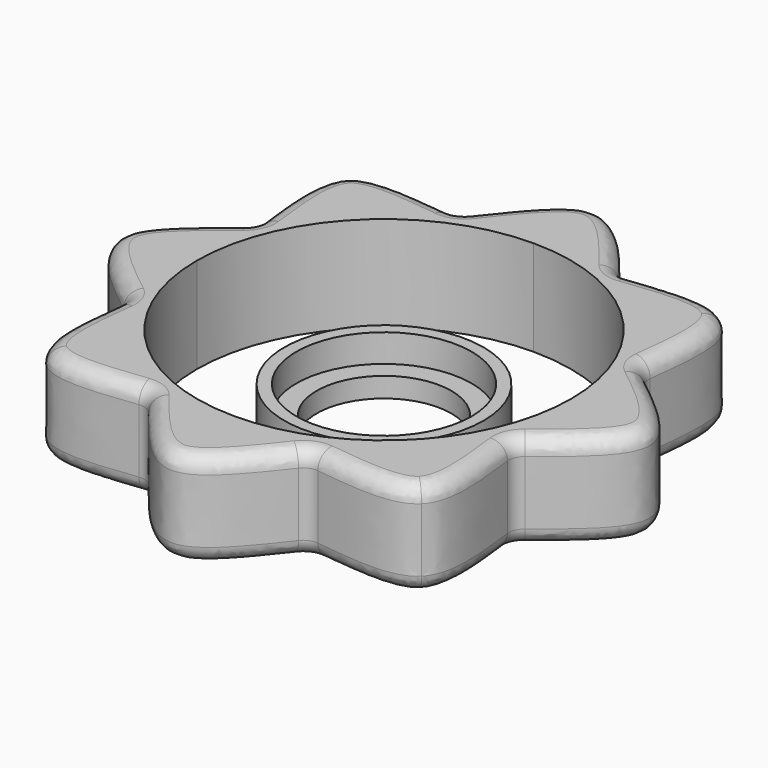
from build123d import *

# Parameters (mm, degrees)
F0_R     = 12.5
F0_R_2   = 11
F0_R_3   = 8.4561388704
F1_DEPTH = 2.5
F2_DEPTH = 12
F3_R     = 2
F4_DEPTH = 6


with BuildPart() as f1:
    # F0 (on Top) → F1 (new body)
    with BuildSketch(Plane.XY):
        Circle(F0_R)
        Circle(F0_R_2, mode=Mode.SUBTRACT)
        Circle(F0_R_2)
        Circle(F0_R_3, mode=Mode.SUBTRACT)
    extrude(amount=F1_DEPTH)

    # F0 (on Top) → F4 (join)
    with BuildSketch(Plane.XY):
        Circle(F0_R)
        Circle(F0_R_2, mode=Mode.SUBTRACT)
    extrude(amount=F4_DEPTH)


with BuildPart() as f2:
    # F0 (on Top) → F2 (new body)
    with BuildSketch(Plane.XY):
        with BuildLine():
            ThreePointArc((-23.5, 0), (-16.6170093579, 16.6170093579), (0, 23.5))
            add(Edge.make_bspline(
                [(-9.1409899994, 24.1728679287), (-6.2252758284, 23.8233956703), (-3.1123029045, 23.4999993166), (0, 23.5)],
                knots=[0.9614800765, 0.9614800765, 0.9614800765, 0.9614800765, 1, 1, 1, 1], degree=3))
            Line((-9.1409899994, 24.1728679287), (-16.656928964, 16.656928964))
            Line((-16.656928964, 16.656928964), (-24.1728340356, 9.1410238925))
            add(Edge.make_bspline(
                [(-23.5, 0), (-23.5, 3.1128517111), (-23.8233482549, 6.2257034223), (-24.1728340356, 9.1410238925)],
                knots=[0.7499999103, 0.7499999103, 0.7499999103, 0.7499999103, 0.7885112511, 0.7885112511, 0.7885112511, 0.7885112511], degree=3))
        make_face()
        with BuildLine():
            add(Edge.make_bspline(
                [(0, -23.5), (-3.1123029045, -23.4999993166), (-6.2252758284, -23.8233956703), (-9.1409899994, -24.1728679287)],
                knots=[0.4999998205, 0.4999998205, 0.4999998205, 0.4999998205, 0.538519744, 0.538519744, 0.538519744, 0.538519744], degree=3))
            ThreePointArc((0, -23.5), (-16.6170093579, -16.6170093579), (-23.5, 0))
            add(Edge.make_bspline(
                [(-24.1728340356, -9.1410238925), (-23.8233482549, -6.2257034223), (-23.5, -3.1128517111), (-23.5, 0)],
                knots=[0.7114885694, 0.7114885694, 0.7114885694, 0.7114885694, 0.7499999103, 0.7499999103, 0.7499999103, 0.7499999103], degree=3))
            Line((-24.1728340356, -9.1410238925), (-16.656928964, -16.656928964))
            Line((-16.656928964, -16.656928964), (-9.1409899994, -24.1728679287))
        make_face()
        with BuildLine():
            ThreePointArc((0, 23.5), (16.6170093579, 16.6170093579), (23.5, 0))
            ThreePointArc((23.5, 0), (16.6170093579, -16.6170093579), (0, -23.5))
            add(Edge.make_bspline(
                [(9.1406888631, -24.173169065), (6.2257012261, -23.8235819149), (3.1131858129, -23.5000006836), (0, -23.5)],
                knots=[0.4614689696, 0.4614689696, 0.4614689696, 0.4614689696, 0.4999998205, 0.4999998205, 0.4999998205, 0.4999998205], degree=3))
            Line((9.1406888631, -24.173169065), (16.656928964, -16.656928964))
            Line((16.656928964, -16.656928964), (24.214399877, -9.0994580511))
            add(Edge.make_bspline(
                [(23.5564548484, 0), (23.5564548484, -3.0980623812), (23.8727564423, -6.1961247624), (24.214399877, -9.0994580511)],
                knots=[0.2499999103, 0.2499999103, 0.2499999103, 0.2499999103, 0.2883282343, 0.2883282343, 0.2883282343, 0.2883282343], degree=3))
            add(Edge.make_bspline(
                [(24.214399877, 9.0994580511), (23.8727564423, 6.1961247624), (23.5564548484, 3.0980623812), (23.5564548484, 0)],
                knots=[0.2116715862, 0.2116715862, 0.2116715862, 0.2116715862, 0.2499999103, 0.2499999103, 0.2499999103, 0.2499999103], degree=3))
            Line((24.214399877, 9.0994580511), (16.656928964, 16.656928964))
            Line((16.656928964, 16.656928964), (9.1406888631, 24.173169065))
            add(Edge.make_bspline(
                [(0, 23.5), (3.1131858129, 23.5000006836), (6.2257012261, 23.8235819149), (9.1406888631, 24.173169065)],
                knots=[0, 0, 0, 0, 0.0385308509, 0.0385308509, 0.0385308509, 0.0385308509], degree=3))
        make_face()
        with BuildLine():
            Line((23.5564548484, 0), (33.3138579281, 0))
            Line((33.3138579281, 0), (24.214399877, 9.0994580511))
            add(Edge.make_bspline(
                [(24.214399877, 9.0994580511), (23.8727564423, 6.1961247624), (23.5564548484, 3.0980623812), (23.5564548484, 0)],
                knots=[0.2116715862, 0.2116715862, 0.2116715862, 0.2116715862, 0.2499999103, 0.2499999103, 0.2499999103, 0.2499999103], degree=3))
        make_face()
        with BuildLine():
            Line((24.214399877, -9.0994580511), (33.3138579281, 0))
            Line((33.3138579281, 0), (23.5564548484, 0))
            add(Edge.make_bspline(
                [(23.5564548484, 0), (23.5564548484, -3.0980623812), (23.8727564423, -6.1961247624), (24.214399877, -9.0994580511)],
                knots=[0.2499999103, 0.2499999103, 0.2499999103, 0.2499999103, 0.2883282343, 0.2883282343, 0.2883282343, 0.2883282343], degree=3))
        make_face()
        with BuildLine():
            add(Edge.make_bspline(
                [(33.3138579281, 0), (33.3138579281, -3.1334505466), (29.1876719761, -6.2669010932), (24.3311990693, -10.0795314392)],
                knots=[0.25, 0.25, 0.25, 0.25, 0.3323011623, 0.3323011623, 0.3323011623, 0.3323011623], degree=3))
            Line((33.3138579281, 0), (24.214399877, -9.0994580511))
            add(Edge.make_bspline(
                [(24.214399877, -9.0994580511), (24.253148452, -9.4287488152), (24.2922230164, -9.755534646), (24.3311990671, -10.0795314387)],
                knots=[0.2883282343, 0.2883282343, 0.2883282343, 0.2883282343, 0.2926753629, 0.2926753629, 0.2926753629, 0.2926753629], degree=3))
        make_face()
        with BuildLine():
            Line((24.214399877, 9.0994580511), (33.3138579281, 0))
            add(Edge.make_bspline(
                [(24.3311990693, 10.0795314392), (29.1876719761, 6.2669010932), (33.3138579281, 3.1334505466), (33.3138579281, 0)],
                knots=[0.1676988377, 0.1676988377, 0.1676988377, 0.1676988377, 0.25, 0.25, 0.25, 0.25], degree=3))
            add(Edge.make_bspline(
                [(24.3311990671, 10.0795314387), (24.2922230164, 9.755534646), (24.253148452, 9.4287488152), (24.214399877, 9.0994580511)],
                knots=[0.2073244576, 0.2073244576, 0.2073244576, 0.2073244576, 0.2116715862, 0.2116715862, 0.2116715862, 0.2116715862], degree=3))
        make_face()
        with BuildLine():
            add(Edge.make_bspline(
                [(16.656928964, 16.656928964), (19.0954369859, 14.2184209422), (21.8116022298, 12.0575701423), (24.3311990693, 10.0795314392)],
                knots=[0.125, 0.125, 0.125, 0.125, 0.1676988377, 0.1676988377, 0.1676988377, 0.1676988377], degree=3))
            Line((16.656928964, 16.656928964), (24.214399877, 9.0994580511))
            add(Edge.make_bspline(
                [(24.3311990671, 10.0795314387), (24.2922230164, 9.755534646), (24.253148452, 9.4287488152), (24.214399877, 9.0994580511)],
                knots=[0.2073244576, 0.2073244576, 0.2073244576, 0.2073244576, 0.2116715862, 0.2116715862, 0.2116715862, 0.2116715862], degree=3))
        make_face()
        with BuildLine():
            Line((24.214399877, -9.0994580511), (16.656928964, -16.656928964))
            add(Edge.make_bspline(
                [(24.3311990693, -10.0795314392), (21.8116022298, -12.0575701423), (19.0954369859, -14.2184209422), (16.656928964, -16.656928964)],
                knots=[0.3323011623, 0.3323011623, 0.3323011623, 0.3323011623, 0.375, 0.375, 0.375, 0.375], degree=3))
            add(Edge.make_bspline(
                [(24.214399877, -9.0994580511), (24.253148452, -9.4287488152), (24.2922230164, -9.755534646), (24.3311990671, -10.0795314387)],
                knots=[0.2883282343, 0.2883282343, 0.2883282343, 0.2883282343, 0.2926753629, 0.2926753629, 0.2926753629, 0.2926753629], degree=3))
        make_face()
        with BuildLine():
            Line((16.656928964, -16.656928964), (23.5564548484, -23.5564548484))
            add(Edge.make_bspline(
                [(24.3311990671, -10.0795314387), (25.0693139916, -16.2152702871), (25.7720984752, -21.3507632582), (23.5564548484, -23.5564548484)],
                knots=[0.2926753629, 0.2926753629, 0.2926753629, 0.2926753629, 0.3749997756, 0.3749997756, 0.3749997756, 0.3749997756], degree=3))
            add(Edge.make_bspline(
                [(24.3311990693, -10.0795314392), (21.8116022298, -12.0575701423), (19.0954369859, -14.2184209422), (16.656928964, -16.656928964)],
                knots=[0.3323011623, 0.3323011623, 0.3323011623, 0.3323011623, 0.375, 0.375, 0.375, 0.375], degree=3))
        make_face()
        with BuildLine():
            add(Edge.make_bspline(
                [(23.5564548484, -23.5564548484), (21.3452428526, -25.7577347135), (16.2272656885, -25.0409215909), (10.1110720196, -24.2910262972)],
                knots=[0.3749997756, 0.3749997756, 0.3749997756, 0.3749997756, 0.4571595268, 0.4571595268, 0.4571595268, 0.4571595268], degree=3))
            Line((23.5564548484, -23.5564548484), (16.656928964, -16.656928964))
            add(Edge.make_bspline(
                [(16.656928964, -16.656928964), (14.2313755557, -19.0824823724), (12.0805370886, -21.782750722), (10.1110720201, -24.2910262998)],
                knots=[0.375, 0.375, 0.375, 0.375, 0.4174719994, 0.4174719994, 0.4174719994, 0.4174719994], degree=3))
        make_face()
        with BuildLine():
            Line((16.656928964, -16.656928964), (9.1406888631, -24.173169065))
            add(Edge.make_bspline(
                [(10.1110720196, -24.2910262972), (9.790265467, -24.2516927939), (9.4667126094, -24.2122682745), (9.1406888631, -24.173169065)],
                knots=[0.4571595268, 0.4571595268, 0.4571595268, 0.4571595268, 0.4614689696, 0.4614689696, 0.4614689696, 0.4614689696], degree=3))
            add(Edge.make_bspline(
                [(16.656928964, -16.656928964), (14.2313755557, -19.0824823724), (12.0805370886, -21.782750722), (10.1110720201, -24.2910262998)],
                knots=[0.375, 0.375, 0.375, 0.375, 0.4174719994, 0.4174719994, 0.4174719994, 0.4174719994], degree=3))
        make_face()
        with BuildLine():
            add(Edge.make_bspline(
                [(23.5564548484, 23.5564548484), (25.7720984752, 21.3507632582), (25.0693139916, 16.2152702871), (24.3311990671, 10.0795314387)],
                knots=[0.1250000449, 0.1250000449, 0.1250000449, 0.1250000449, 0.2073244576, 0.2073244576, 0.2073244576, 0.2073244576], degree=3))
            Line((23.5564548484, 23.5564548484), (16.656928964, 16.656928964))
            add(Edge.make_bspline(
                [(16.656928964, 16.656928964), (19.0954369859, 14.2184209422), (21.8116022298, 12.0575701423), (24.3311990693, 10.0795314392)],
                knots=[0.125, 0.125, 0.125, 0.125, 0.1676988377, 0.1676988377, 0.1676988377, 0.1676988377], degree=3))
        make_face()
        with BuildLine():
            Line((16.656928964, 16.656928964), (23.5564548484, 23.5564548484))
            add(Edge.make_bspline(
                [(10.1110720196, 24.2910262972), (16.2272656885, 25.0409215909), (21.3452428526, 25.7577347135), (23.5564548484, 23.5564548484)],
                knots=[0.0428402937, 0.0428402937, 0.0428402937, 0.0428402937, 0.1250000449, 0.1250000449, 0.1250000449, 0.1250000449], degree=3))
            add(Edge.make_bspline(
                [(10.1110720201, 24.2910262998), (12.0805370886, 21.782750722), (14.2313755557, 19.0824823724), (16.656928964, 16.656928964)],
                knots=[0.0825280006, 0.0825280006, 0.0825280006, 0.0825280006, 0.125, 0.125, 0.125, 0.125], degree=3))
        make_face()
        with BuildLine():
            add(Edge.make_bspline(
                [(9.1406888631, 24.173169065), (9.4667126094, 24.2122682745), (9.790265467, 24.2516927939), (10.1110720196, 24.2910262972)],
                knots=[0.0385308509, 0.0385308509, 0.0385308509, 0.0385308509, 0.0428402937, 0.0428402937, 0.0428402937, 0.0428402937], degree=3))
            Line((9.1406888631, 24.173169065), (16.656928964, 16.656928964))
            add(Edge.make_bspline(
                [(10.1110720201, 24.2910262998), (12.0805370886, 21.782750722), (14.2313755557, 19.0824823724), (16.656928964, 16.656928964)],
                knots=[0.0825280006, 0.0825280006, 0.0825280006, 0.0825280006, 0.125, 0.125, 0.125, 0.125], degree=3))
        make_face()
        with BuildLine():
            add(Edge.make_bspline(
                [(0, 33.3138579281), (3.1420869556, 33.3138579281), (6.2841739112, 29.164895463), (10.1110720201, 24.2910262998)],
                knots=[0, 0, 0, 0, 0.0825280006, 0.0825280006, 0.0825280006, 0.0825280006], degree=3))
            Line((0, 33.3138579281), (9.1406888631, 24.173169065))
            add(Edge.make_bspline(
                [(9.1406888631, 24.173169065), (9.4667126094, 24.2122682745), (9.790265467, 24.2516927939), (10.1110720196, 24.2910262972)],
                knots=[0.0385308509, 0.0385308509, 0.0385308509, 0.0385308509, 0.0428402937, 0.0428402937, 0.0428402937, 0.0428402937], degree=3))
        make_face()
        with BuildLine():
            add(Edge.make_bspline(
                [(-9.1409899994, 24.1728679287), (-6.2252758284, 23.8233956703), (-3.1123029045, 23.4999993166), (0, 23.5)],
                knots=[0.9614800765, 0.9614800765, 0.9614800765, 0.9614800765, 1, 1, 1, 1], degree=3))
            Line((0, 23.5), (0, 33.3138579281))
            Line((0, 33.3138579281), (-9.1409899994, 24.1728679287))
        make_face()
        with BuildLine():
            Line((0, 33.3138579281), (0, 23.5))
            add(Edge.make_bspline(
                [(0, 23.5), (3.1131858129, 23.5000006836), (6.2257012261, 23.8235819149), (9.1406888631, 24.173169065)],
                knots=[0, 0, 0, 0, 0.0385308509, 0.0385308509, 0.0385308509, 0.0385308509], degree=3))
            Line((9.1406888631, 24.173169065), (0, 33.3138579281))
        make_face()
        with BuildLine():
            Line((-9.1409899994, 24.1728679287), (0, 33.3138579281))
            add(Edge.make_bspline(
                [(-10.1113617747, 24.2906572738), (-6.2843325131, 29.1646860348), (-3.1421662565, 33.3138579281), (0, 33.3138579281)],
                knots=[0.9174699166, 0.9174699166, 0.9174699166, 0.9174699166, 1, 1, 1, 1], degree=3))
            add(Edge.make_bspline(
                [(-10.1113617741, 24.2906572713), (-9.7905551459, 24.2513452368), (-9.4670056585, 24.2119435794), (-9.1409899994, 24.1728679287)],
                knots=[0.9571730363, 0.9571730363, 0.9571730363, 0.9571730363, 0.9614800765, 0.9614800765, 0.9614800765, 0.9614800765], degree=3))
        make_face()
        with BuildLine():
            Line((-16.656928964, 16.656928964), (-9.1409899994, 24.1728679287))
            add(Edge.make_bspline(
                [(-10.1113617741, 24.2906572713), (-9.7905551459, 24.2513452368), (-9.4670056585, 24.2119435794), (-9.1409899994, 24.1728679287)],
                knots=[0.9571730363, 0.9571730363, 0.9571730363, 0.9571730363, 0.9614800765, 0.9614800765, 0.9614800765, 0.9614800765], degree=3))
            add(Edge.make_bspline(
                [(-16.656928964, 16.656928964), (-14.2314945071, 19.082363421), (-12.0807480475, 21.7824858753), (-10.1113617747, 24.2906572738)],
                knots=[0.875, 0.875, 0.875, 0.875, 0.9174699166, 0.9174699166, 0.9174699166, 0.9174699166], degree=3))
        make_face()
        with BuildLine():
            Line((-16.656928964, 16.656928964), (-23.5564548484, 23.5564548484))
            add(Edge.make_bspline(
                [(-24.2906447975, 10.1113715684), (-25.0409807835, 16.2330345897), (-25.7589906868, 21.3545821099), (-23.5564548484, 23.5564548484)],
                knots=[0.7928178581, 0.7928178581, 0.7928178581, 0.7928178581, 0.8749999551, 0.8749999551, 0.8749999551, 0.8749999551], degree=3))
            add(Edge.make_bspline(
                [(-24.2906448, 10.111371569), (-21.782476923, 12.0807551784), (-19.0823594002, 14.2314985279), (-16.656928964, 16.656928964)],
                knots=[0.8325301538, 0.8325301538, 0.8325301538, 0.8325301538, 0.875, 0.875, 0.875, 0.875], degree=3))
        make_face()
        with BuildLine():
            add(Edge.make_bspline(
                [(-23.5564548484, 23.5564548484), (-21.3541606416, 25.7580860283), (-16.2319614609, 25.0406830033), (-10.1113617741, 24.2906572713)],
                knots=[0.8749999551, 0.8749999551, 0.8749999551, 0.8749999551, 0.9571730363, 0.9571730363, 0.9571730363, 0.9571730363], degree=3))
            Line((-23.5564548484, 23.5564548484), (-16.656928964, 16.656928964))
            add(Edge.make_bspline(
                [(-16.656928964, 16.656928964), (-14.2314945071, 19.082363421), (-12.0807480475, 21.7824858753), (-10.1113617747, 24.2906572738)],
                knots=[0.875, 0.875, 0.875, 0.875, 0.9174699166, 0.9174699166, 0.9174699166, 0.9174699166], degree=3))
        make_face()
        with BuildLine():
            add(Edge.make_bspline(
                [(-23.5564548484, -23.5564548484), (-25.7589906868, -21.3545821099), (-25.0409807835, -16.2330345897), (-24.2906447975, -10.1113715684)],
                knots=[0.6249998654, 0.6249998654, 0.6249998654, 0.6249998654, 0.7071819624, 0.7071819624, 0.7071819624, 0.7071819624], degree=3))
            Line((-23.5564548484, -23.5564548484), (-16.656928964, -16.656928964))
            add(Edge.make_bspline(
                [(-16.656928964, -16.656928964), (-19.0823594002, -14.2314985279), (-21.782476923, -12.0807551784), (-24.2906448, -10.111371569)],
                knots=[0.625, 0.625, 0.625, 0.625, 0.6674698462, 0.6674698462, 0.6674698462, 0.6674698462], degree=3))
        make_face()
        with BuildLine():
            Line((-16.656928964, -16.656928964), (-23.5564548484, -23.5564548484))
            add(Edge.make_bspline(
                [(-10.1113617741, -24.2906572713), (-16.2319614609, -25.0406830033), (-21.3541606416, -25.7580860283), (-23.5564548484, -23.5564548484)],
                knots=[0.5428267842, 0.5428267842, 0.5428267842, 0.5428267842, 0.6249998654, 0.6249998654, 0.6249998654, 0.6249998654], degree=3))
            add(Edge.make_bspline(
                [(-10.1113617747, -24.2906572738), (-12.0807480475, -21.7824858753), (-14.2314945071, -19.082363421), (-16.656928964, -16.656928964)],
                knots=[0.5825300834, 0.5825300834, 0.5825300834, 0.5825300834, 0.625, 0.625, 0.625, 0.625], degree=3))
        make_face()
        with BuildLine():
            Line((-24.1728340356, -9.1410238925), (-33.3138579281, 0))
            add(Edge.make_bspline(
                [(-24.2906448, -10.111371569), (-29.1646789557, -6.2843378741), (-33.3138579281, -3.142168937), (-33.3138579281, 0)],
                knots=[0.6674698462, 0.6674698462, 0.6674698462, 0.6674698462, 0.75, 0.75, 0.75, 0.75], degree=3))
            add(Edge.make_bspline(
                [(-24.2906447975, -10.1113715684), (-24.2513247716, -9.7905766807), (-24.2119159752, -9.4670353777), (-24.1728340356, -9.1410238925)],
                knots=[0.7071819624, 0.7071819624, 0.7071819624, 0.7071819624, 0.7114885694, 0.7114885694, 0.7114885694, 0.7114885694], degree=3))
        make_face()
        with BuildLine():
            add(Edge.make_bspline(
                [(-24.1728340356, -9.1410238925), (-23.8233482549, -6.2257034223), (-23.5, -3.1128517111), (-23.5, 0)],
                knots=[0.7114885694, 0.7114885694, 0.7114885694, 0.7114885694, 0.7499999103, 0.7499999103, 0.7499999103, 0.7499999103], degree=3))
            Line((-23.5, 0), (-33.3138579281, 0))
            Line((-33.3138579281, 0), (-24.1728340356, -9.1410238925))
        make_face()
        with BuildLine():
            Line((-33.3138579281, 0), (-23.5, 0))
            add(Edge.make_bspline(
                [(-23.5, 0), (-23.5, 3.1128517111), (-23.8233482549, 6.2257034223), (-24.1728340356, 9.1410238925)],
                knots=[0.7499999103, 0.7499999103, 0.7499999103, 0.7499999103, 0.7885112511, 0.7885112511, 0.7885112511, 0.7885112511], degree=3))
            Line((-24.1728340356, 9.1410238925), (-33.3138579281, 0))
        make_face()
        with BuildLine():
            add(Edge.make_bspline(
                [(-33.3138579281, 0), (-33.3138579281, 3.142168937), (-29.1646789557, 6.2843378741), (-24.2906448, 10.111371569)],
                knots=[0.75, 0.75, 0.75, 0.75, 0.8325301538, 0.8325301538, 0.8325301538, 0.8325301538], degree=3))
            Line((-33.3138579281, 0), (-24.1728340356, 9.1410238925))
            add(Edge.make_bspline(
                [(-24.1728340356, 9.1410238925), (-24.2119159752, 9.4670353777), (-24.2513247716, 9.7905766807), (-24.2906447975, 10.1113715684)],
                knots=[0.7885112511, 0.7885112511, 0.7885112511, 0.7885112511, 0.7928178581, 0.7928178581, 0.7928178581, 0.7928178581], degree=3))
        make_face()
        with BuildLine():
            add(Edge.make_bspline(
                [(-24.1728340356, 9.1410238925), (-24.2119159752, 9.4670353777), (-24.2513247716, 9.7905766807), (-24.2906447975, 10.1113715684)],
                knots=[0.7885112511, 0.7885112511, 0.7885112511, 0.7885112511, 0.7928178581, 0.7928178581, 0.7928178581, 0.7928178581], degree=3))
            Line((-24.1728340356, 9.1410238925), (-16.656928964, 16.656928964))
            add(Edge.make_bspline(
                [(-24.2906448, 10.111371569), (-21.782476923, 12.0807551784), (-19.0823594002, 14.2314985279), (-16.656928964, 16.656928964)],
                knots=[0.8325301538, 0.8325301538, 0.8325301538, 0.8325301538, 0.875, 0.875, 0.875, 0.875], degree=3))
        make_face()
        with BuildLine():
            Line((-16.656928964, -16.656928964), (-24.1728340356, -9.1410238925))
            add(Edge.make_bspline(
                [(-24.2906447975, -10.1113715684), (-24.2513247716, -9.7905766807), (-24.2119159752, -9.4670353777), (-24.1728340356, -9.1410238925)],
                knots=[0.7071819624, 0.7071819624, 0.7071819624, 0.7071819624, 0.7114885694, 0.7114885694, 0.7114885694, 0.7114885694], degree=3))
            add(Edge.make_bspline(
                [(-16.656928964, -16.656928964), (-19.0823594002, -14.2314985279), (-21.782476923, -12.0807551784), (-24.2906448, -10.111371569)],
                knots=[0.625, 0.625, 0.625, 0.625, 0.6674698462, 0.6674698462, 0.6674698462, 0.6674698462], degree=3))
        make_face()
        with BuildLine():
            add(Edge.make_bspline(
                [(-9.1409899994, -24.1728679287), (-9.4670056585, -24.2119435794), (-9.7905551459, -24.2513452368), (-10.1113617741, -24.2906572713)],
                knots=[0.538519744, 0.538519744, 0.538519744, 0.538519744, 0.5428267842, 0.5428267842, 0.5428267842, 0.5428267842], degree=3))
            Line((-9.1409899994, -24.1728679287), (-16.656928964, -16.656928964))
            add(Edge.make_bspline(
                [(-10.1113617747, -24.2906572738), (-12.0807480475, -21.7824858753), (-14.2314945071, -19.082363421), (-16.656928964, -16.656928964)],
                knots=[0.5825300834, 0.5825300834, 0.5825300834, 0.5825300834, 0.625, 0.625, 0.625, 0.625], degree=3))
        make_face()
        with BuildLine():
            Line((0, -33.3138579281), (0, -23.5))
            add(Edge.make_bspline(
                [(0, -23.5), (-3.1123029045, -23.4999993166), (-6.2252758284, -23.8233956703), (-9.1409899994, -24.1728679287)],
                knots=[0.4999998205, 0.4999998205, 0.4999998205, 0.4999998205, 0.538519744, 0.538519744, 0.538519744, 0.538519744], degree=3))
            Line((-9.1409899994, -24.1728679287), (0, -33.3138579281))
        make_face()
        with BuildLine():
            add(Edge.make_bspline(
                [(0, -33.3138579281), (-3.1421662565, -33.3138579281), (-6.2843325131, -29.1646860348), (-10.1113617747, -24.2906572738)],
                knots=[0.5, 0.5, 0.5, 0.5, 0.5825300834, 0.5825300834, 0.5825300834, 0.5825300834], degree=3))
            Line((0, -33.3138579281), (-9.1409899994, -24.1728679287))
            add(Edge.make_bspline(
                [(-9.1409899994, -24.1728679287), (-9.4670056585, -24.2119435794), (-9.7905551459, -24.2513452368), (-10.1113617741, -24.2906572713)],
                knots=[0.538519744, 0.538519744, 0.538519744, 0.538519744, 0.5428267842, 0.5428267842, 0.5428267842, 0.5428267842], degree=3))
        make_face()
        with BuildLine():
            Line((9.1406888631, -24.173169065), (0, -33.3138579281))
            add(Edge.make_bspline(
                [(10.1110720201, -24.2910262998), (6.2841739112, -29.164895463), (3.1420869556, -33.3138579281), (0, -33.3138579281)],
                knots=[0.4174719994, 0.4174719994, 0.4174719994, 0.4174719994, 0.5, 0.5, 0.5, 0.5], degree=3))
            add(Edge.make_bspline(
                [(10.1110720196, -24.2910262972), (9.790265467, -24.2516927939), (9.4667126094, -24.2122682745), (9.1406888631, -24.173169065)],
                knots=[0.4571595268, 0.4571595268, 0.4571595268, 0.4571595268, 0.4614689696, 0.4614689696, 0.4614689696, 0.4614689696], degree=3))
        make_face()
        with BuildLine():
            add(Edge.make_bspline(
                [(9.1406888631, -24.173169065), (6.2257012261, -23.8235819149), (3.1131858129, -23.5000006836), (0, -23.5)],
                knots=[0.4614689696, 0.4614689696, 0.4614689696, 0.4614689696, 0.4999998205, 0.4999998205, 0.4999998205, 0.4999998205], degree=3))
            Line((0, -23.5), (0, -33.3138579281))
            Line((0, -33.3138579281), (9.1406888631, -24.173169065))
        make_face()
    extrude(amount=F2_DEPTH)

    # F3
    f3_edges = [f2.edges().sort_by_distance(p)[0] for p in [
        (33.313858, 0, 0),
        (23.569227, -23.543675, 0),
        (24.331199, -10.079531, 6),
        (10.111072, -24.291026, 6),
        (-10.111362, -24.290657, 6),
        (-33.313858, 0, 0),
        (-24.290645, 10.111372, 6),
        (-24.290645, -10.111372, 6),
        (-10.111362, 24.290657, 6),
        (10.111072, 24.291026, 6),
        (24.331199, 10.079531, 6),
        (-23.556561, 23.556348, 12),
        (-33.313858, 0, 12),
        (-23.556817, -23.556092, 0),
        (-23.556817, -23.556092, 12),
        (-0.000119, -33.313858, 0),
        (-0.000119, -33.313858, 12),
        (23.563094, -23.549828, 12),
        (33.313858, 0, 12),
        (23.563094, 23.549828, 0),
        (23.563094, 23.549828, 12),
        (-0.000119, 33.313858, 0),
        (-0.000119, 33.313858, 12),
        (-23.556817, 23.556092, 0),
    ]]
    fillet(f3_edges, radius=F3_R)


solid = Compound([f1.part, f2.part])
